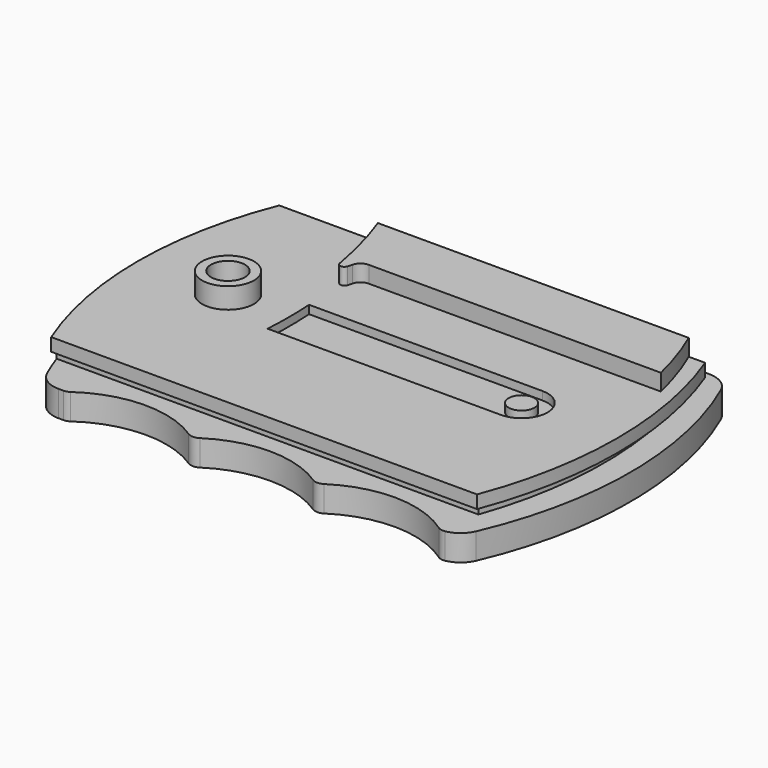
from build123d import *

# Parameters (mm, degrees)
F1_DEPTH     = 6.35
F2_R         = 3.175
F3_R         = 3.175
F4_DEPTH     = 2.54
F6_DEPTH     = 2.032
F7_T1_DEPTH  = 7.9826274972
F8_R         = 3.175
F9_R         = 2.0828
F10_DEPTH    = 4.7625
F12_DEPTH    = 1.016
F13_R        = 3.17499
F14_R        = 1.5875
F15_DEPTH    = 1.016
F19_DEPTH    = 6.351
F20_T1_DEPTH = 9.3839178422
F20_T3_DEPTH = 10.5760872304
F20_T5_DEPTH = 8.4107682306
F25_DEPTH    = 63.5


# Not quite as in the source:
# - a fillet or chamfer that OpenCascade refuses, or shapes differently, is made with other operations: its cross-section is extruded or revolved along the edge and cut away or added
# - a fillet or chamfer is up to 0.001 mm smaller than in the source, because OpenCascade refuses the exact size
# - a feature of the source that left no trace in its solid (it failed there, or was rolled back) is left out


with BuildPart() as f1:
    # F0 (on Top) → F1 (new body)
    with BuildSketch(Plane.XY):
        with BuildLine():
            ThreePointArc((25.4, -20.6375), (30.1625, 0), (25.4, 20.6375))
            Line((25.4, 20.6375), (-25.4, 20.6375))
            ThreePointArc((-25.4, 20.6375), (-30.1625, 0), (-25.4, -20.6375))
            Line((-25.4, -20.6375), (25.4, -20.6375))
        make_face()
    extrude(amount=F1_DEPTH)

    # F2
    f2_edges = [f1.edges().sort_by_distance(p)[0] for p in [
        (-25.4, 20.6375, 3.175),
        (-25.4, -20.6375, 3.175),
        (25.4, -20.6375, 3.175),
        (25.4, 20.6375, 3.175),
    ]]
    fillet(f2_edges, radius=F2_R)

    # F3 (on face) → F4 (join)
    with BuildSketch(Plane.XY.offset(6.35)):
        with Locations((-19.1135, 0)):
            Circle(F3_R)
    extrude(amount=F4_DEPTH)

    # F5 (on face) → F6 (join)
    with BuildSketch(Plane.XY.offset(6.35)):
        with BuildLine():
            ThreePointArc((25.7962114887, 10.16), (24.151933107, 15.5254784859), (21.8369283945, 20.6375))
            Line((21.8369283945, 20.6375), (-16.002, 20.6375))
            ThreePointArc((-16.002, 20.6375), (-13.4865218815, 13.6398781095), (-12.0195455914, 6.35))
            Line((-12.0195455914, 6.35), (-11.2165052403, 9.2309969527))
            ThreePointArc((-11.2165052403, 9.2309969527), (-10.7612010879, 9.9014262529), (-9.9931405857, 10.16))
            Line((-9.9931405857, 10.16), (25.7962114887, 10.16))
        make_face()
    extrude(amount=F6_DEPTH)

    # F7: fillet of radius 0.508 on 1 edges, made by hand

    # F7_s2 → F7_t1 (cut)
    with BuildSketch(Plane.XY.offset(6.35)):
        with BuildLine():
            ThreePointArc((-12.3702984959, 8.6923219718), (-11.8951499479, 8.2718785653), (-11.3804445383, 8.6428464104))
            Line((-11.3804445383, 8.6428464104), (-12.0195455914, 6.35))
            ThreePointArc((-12.0195455914, 6.35), (-12.1812694874, 7.523205399), (-12.3702984959, 8.6923219718))
        make_face()
    extrude(amount=F7_T1_DEPTH, mode=Mode.SUBTRACT)

    # F8
    f8_edges = [f1.edges().sort_by_distance(p)[0] for p in [
        (21.836928, 20.6375, 7.366),
    ]]
    fillet(f8_edges, radius=F8_R)

    # F9 (on face) → F10 (cut)
    with BuildSketch(Plane.XY.offset(8.89)):
        with Locations((-19.1135, 0)):
            Circle(F9_R)
    extrude(amount=-F10_DEPTH, mode=Mode.SUBTRACT)

    # F11 (on face) → F12 (cut)
    with BuildSketch(Plane.XY.offset(6.35)):
        with BuildLine():
            ThreePointArc((-11.7204239002, 3.175), (-11.6211080672, 0), (-11.7204239002, -3.175))
            Line((-11.7204239002, -3.175), (20.0295760998, -3.175))
            Line((20.0295760998, -3.175), (20.0295760998, 3.175))
            Line((20.0295760998, 3.175), (-11.7204239002, 3.175))
        make_face()
    extrude(amount=-F12_DEPTH, mode=Mode.SUBTRACT)

    # F13 (radius 3.175 in the source; OpenCascade refuses exactly that, so slightly less here)
    f13_edges = [f1.edges().sort_by_distance(p)[0] for p in [
        (20.029576, 3.175, 5.842),
        (20.029576, -3.175, 5.842),
    ]]
    fillet(f13_edges, radius=F13_R)

    # F14 (on face) → F15 (join, through all)
    with BuildSketch(Plane.XY.offset(5.334)):
        with Locations((16.8545760998, 0)):
            Circle(F14_R)
    extrude(amount=F15_DEPTH)

    # F18 (on face) → F19 (cut, through all)
    with BuildSketch(Plane.XY.offset(6.35)):
        with BuildLine():
            Line((8.1267993519, -20.6375), (23.3667993519, -20.6375))
            ThreePointArc((23.3667993519, -20.6375), (15.7467993519, -18.0975), (8.1267993519, -20.6375))
        make_face()
        with BuildLine():
            Line((-7.1132006481, -20.6375), (8.1267993519, -20.6375))
            ThreePointArc((8.1267993519, -20.6375), (0.5067993519, -18.0975), (-7.1132006481, -20.6375))
        make_face()
        with BuildLine():
            Line((-22.3532006481, -20.6375), (-7.1132006481, -20.6375))
            ThreePointArc((-7.1132006481, -20.6375), (-14.7332006481, -18.0975), (-22.3532006481, -20.6375))
        make_face()
    extrude(amount=-F19_DEPTH, mode=Mode.SUBTRACT)

    # F20: fillet of radius 1.27 on 4 edges, made by hand

    # F20_s2 → F20_t1 (cut)
    with BuildSketch(Plane.XY.offset(-1.5169589211)):
        with BuildLine():
            ThreePointArc((23.9708158767, -20.5796179073), (23.4664541239, -20.5753299276), (23.0035373612, -20.3750620187))
            Line((23.0035373612, -20.3750620187), (22.9890237709, -20.3959070588))
            ThreePointArc((22.9890237709, -20.3959070588), (23.1714765643, -20.5252240374), (23.3515593519, -20.65782))
            Line((23.3515593519, -20.65782), (23.3667993519, -20.6629))
            ThreePointArc((23.3667993519, -20.6629), (23.6726182662, -20.648255005), (23.9756478567, -20.6045540651))
            Line((23.9756478567, -20.6045540651), (23.9708158767, -20.5796179073))
        make_face()
    extrude(amount=F20_T1_DEPTH, mode=Mode.SUBTRACT)

    # F20_s4 → F20_t3 (cut)
    with BuildSketch(Plane.XY.offset(-2.1130436152)):
        with BuildLine():
            ThreePointArc((8.8195315833, -20.1532329387), (8.1267993519, -20.3587978512), (7.4340671204, -20.1532329387))
            Line((7.4340671204, -20.1532329387), (7.4202124758, -20.1745216404))
            ThreePointArc((7.4202124758, -20.1745216404), (7.7699369678, -20.410377341), (8.1115593519, -20.65782))
            Line((8.1115593519, -20.65782), (8.1420393519, -20.65782))
            ThreePointArc((8.1420393519, -20.65782), (8.4836617359, -20.410377341), (8.8333862279, -20.1745216404))
            Line((8.8333862279, -20.1745216404), (8.8195315833, -20.1532329387))
        make_face()
        with BuildLine():
            ThreePointArc((-6.4204684167, -20.1532329387), (-7.1132006481, -20.3587978512), (-7.8059328796, -20.1532329387))
            Line((-7.8059328796, -20.1532329387), (-7.8197875242, -20.1745216404))
            ThreePointArc((-7.8197875242, -20.1745216404), (-7.4700630322, -20.410377341), (-7.1284406481, -20.65782))
            Line((-7.1284406481, -20.65782), (-7.0979606481, -20.65782))
            ThreePointArc((-7.0979606481, -20.65782), (-6.7563382641, -20.410377341), (-6.4066137721, -20.1745216404))
            Line((-6.4066137721, -20.1745216404), (-6.4204684167, -20.1532329387))
        make_face()
    extrude(amount=F20_T3_DEPTH, mode=Mode.SUBTRACT)

    # F20_s6 → F20_t5 (cut)
    with BuildSketch(Plane.XY.offset(-1.0303841153)):
        with BuildLine():
            ThreePointArc((-22.0351532703, -20.4066892562), (-22.382433504, -20.5784970549), (-22.7653542821, -20.6376))
            Line((-22.7653542821, -20.6376), (-22.7653542821, -20.663))
            ThreePointArc((-22.7653542821, -20.663), (-22.5592774651, -20.6629), (-22.3532006481, -20.6629))
            Line((-22.3532006481, -20.6629), (-22.3379606481, -20.65782))
            ThreePointArc((-22.3379606481, -20.65782), (-22.1801756491, -20.5413775117), (-22.0205492501, -20.4274710413))
            Line((-22.0205492501, -20.4274710413), (-22.0351532703, -20.4066892562))
        make_face()
    extrude(amount=F20_T5_DEPTH, mode=Mode.SUBTRACT)

    # F21 (on Front) → F23 (revolve, cut)
    with BuildSketch(Plane.XZ):
        Polygon((26.9875, 4.7625), (26.9875, 3.175), (30.1625, 3.175), (30.1625, 6.35), (28.575, 6.35), (28.575, 4.7625), align=None)
    revolve(axis=Axis((-20.6375, 0, 8.7874885648), (0, 0, 1)), mode=Mode.SUBTRACT)

    # F24 (on Right) → F25 (cut, symmetric)
    with BuildSketch(Plane.YZ):
        Polygon((15.875, 3.175), (20.6375, 3.175), (20.6375, 8.382), (17.4625, 8.382), (17.4625, 4.7625), (15.875, 4.7625), align=None)
        Polygon((-15.875, 4.7625), (-17.4625, 4.7625), (-17.4625, 8.382), (-20.6375, 8.382), (-20.6375, 3.175), (-15.875, 3.175), align=None)
    extrude(amount=F25_DEPTH, both=True, mode=Mode.SUBTRACT)


solid = f1.part
